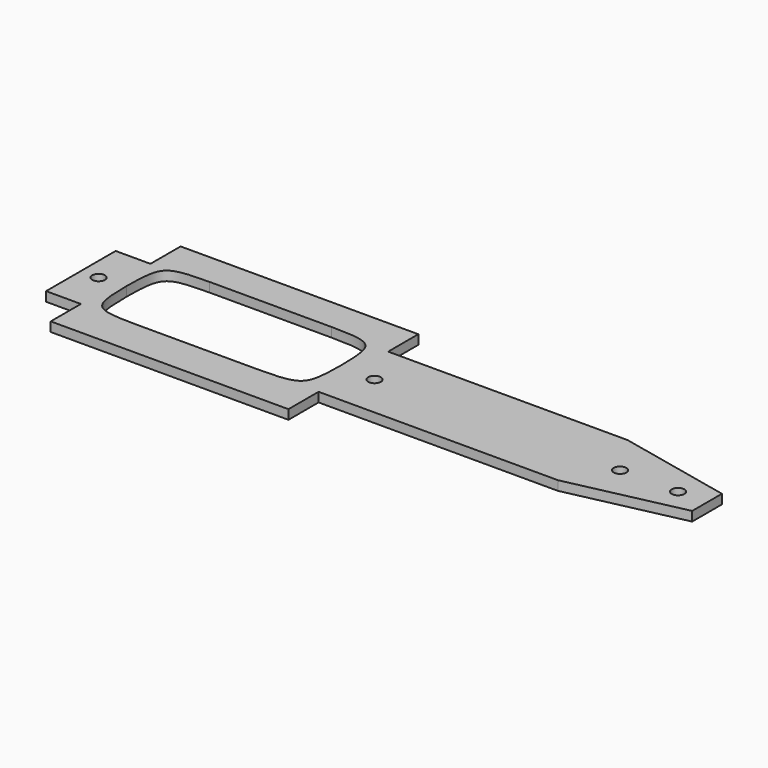
from build123d import *

# Parameters (mm, degrees)
F0_W        = 77.47
F0_H        = 19.05
F0_R        = 1.3890625
F0_W_2      = 52.07
F0_H_2      = 8.255
F0_W_3      = 7.62
F1_DEPTH    = 2.0574
F2_R        = 1.3890625
F2_W        = 46.99
F2_H        = 20.1539304107
F3_DEPTH    = 25.4
F4_T1_DEPTH = 2.0574


# Not quite as in the source:
# - a fillet or chamfer that OpenCascade refuses, or shapes differently, is made with other operations: its cross-section is extruded or revolved along the edge and cut away or added


with BuildPart() as f1:
    # F0 (on Top) → F1 (new body)
    with BuildSketch(Plane.XY):
        with Locations((29.845, 0)):
            Rectangle(F0_W, F0_H)
        with Locations((-4.2449974041, 0)):
            Circle(F0_R, mode=Mode.SUBTRACT)
        with Locations((-34.925, -13.6525)):
            Rectangle(F0_W_2, F0_H_2)
        with Locations((-34.925, 0)):
            Rectangle(F0_W_2, F0_H)
        with Locations((-64.77, 0)):
            Rectangle(F0_W_3, F0_H)
        with Locations((-64.6969974041, 0)):
            Circle(F0_R, mode=Mode.SUBTRACT)
        with Locations((-34.925, 13.6525)):
            Rectangle(F0_W_2, F0_H_2)
    extrude(amount=F1_DEPTH)

    # F2 (on face) → F3 (cut)
    with BuildSketch(Plane.XY.offset(2.0574)):
        Polygon((43.5640997417, 9.525), (68.58, 4.0749409236), (68.58, 9.525), align=None)
        Polygon((68.58, -9.525), (68.58, -4.0749409236), (43.5640997417, -9.525), align=None)
        with Locations((49.53, 0)):
            Circle(F2_R)
        with Locations((62.23, 0)):
            Circle(F2_R)
        with Locations((-35.5063436133, 0.5281241611)):
            Rectangle(F2_W, F2_H)
    extrude(amount=-F3_DEPTH, mode=Mode.SUBTRACT)

    # F4: fillet of radius 10.16 on 4 edges, made by hand

    # F4_s2 → F4_t1 (join)
    with BuildSketch(Plane.XY):
        with BuildLine():
            add(Edge.make_bspline(
                [(-22.1713436133, 10.6050893664), (-12.0113436133, 10.6050893664), (-12.0113436133, 0.4450893664)],
                knots=[0, 0, 0, 1, 1, 1], degree=2, weights=[1, 2.3333333333, 1]))
            Line((-12.0113436133, 0.4450893664), (-12.0113436133, 10.6050893664))
            Line((-12.0113436133, 10.6050893664), (-22.1713436133, 10.6050893664))
        make_face()
        with BuildLine():
            add(Edge.make_bspline(
                [(-48.8413436133, 10.6050893664), (-59.0013436133, 10.6050893664), (-59.0013436133, 0.4450893664)],
                knots=[0, 0, 0, 1, 1, 1], degree=2, weights=[1, 2.3333333333, 1]))
            Line((-59.0013436133, 0.4450893664), (-59.0013436133, 10.6050893664))
            Line((-59.0013436133, 10.6050893664), (-48.8413436133, 10.6050893664))
        make_face()
        with BuildLine():
            add(Edge.make_bspline(
                [(-59.0013436133, 0.6111589557), (-59.0013436133, -9.5488410443), (-48.8413436133, -9.5488410443)],
                knots=[0, 0, 0, 1, 1, 1], degree=2, weights=[1, 2.3333333333, 1]))
            Line((-48.8413436133, -9.5488410443), (-59.0013436133, -9.5488410443))
            Line((-59.0013436133, -9.5488410443), (-59.0013436133, 0.6111589557))
        make_face()
        with BuildLine():
            add(Edge.make_bspline(
                [(-22.1713436133, -9.5488410443), (-12.0113436133, -9.5488410443), (-12.0113436133, 0.6111589557)],
                knots=[0, 0, 0, 1, 1, 1], degree=2, weights=[1, 2.3333333333, 1]))
            Line((-12.0113436133, 0.6111589557), (-12.0113436133, -9.5488410443))
            Line((-12.0113436133, -9.5488410443), (-22.1713436133, -9.5488410443))
        make_face()
    extrude(amount=F4_T1_DEPTH)


solid = f1.part
